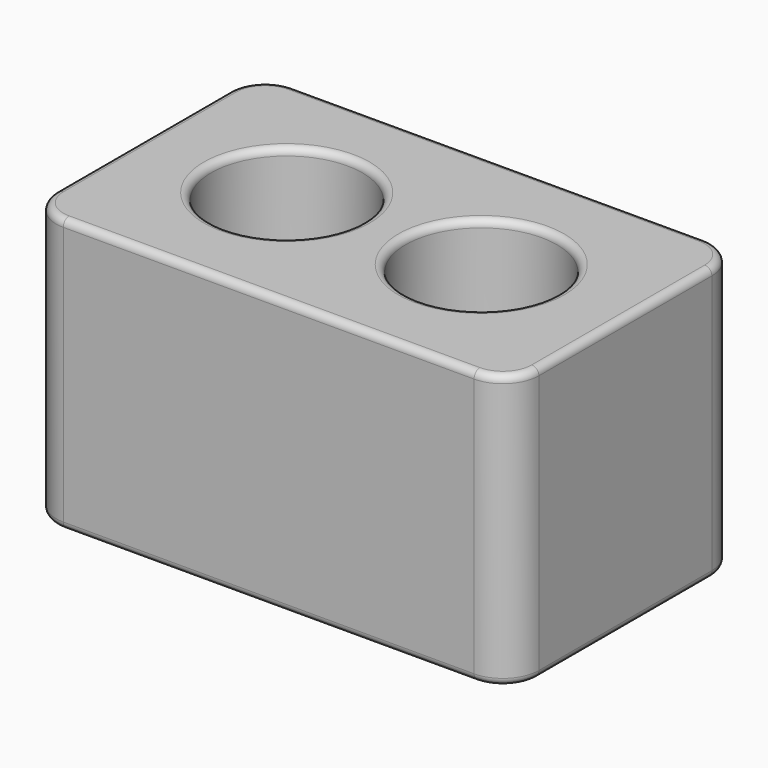
from build123d import *

# Parameters (mm, degrees)
F0_W         = 67
F0_H         = 40
F0_R         = 10.5
F1_DEPTH     = 36
F2_W         = 67
F2_H         = 40
F3_DEPTH     = 2
F4_R         = 1
F5_T1_DEPTH  = 38
F5_T4_ANGLE  = 90
F5_T6_ANGLE  = 90
F5_T8_ANGLE  = 90
F5_T10_ANGLE = 90
F5_T12_ANGLE = 90
F5_T14_ANGLE = 90
F5_T16_ANGLE = 90
F5_T18_ANGLE = 90


# Not quite as in the source:
# - a fillet or chamfer that OpenCascade refuses, or shapes differently, is made with other operations: its cross-section is extruded or revolved along the edge and cut away or added


with BuildPart() as f1:
    # F0 (on Top) → F1 (new body)
    with BuildSketch(Plane.XY):
        Rectangle(F0_W, F0_H)
        with Locations((-13.5, 0)):
            Circle(F0_R, mode=Mode.SUBTRACT)
        with Locations((13.5, 0)):
            Circle(F0_R, mode=Mode.SUBTRACT)
    extrude(amount=F1_DEPTH)

    # F2 (on face) → F3 (join)
    with BuildSketch(Plane(origin=(0, 0, 0), x_dir=(1, 0, 0), z_dir=(0, 0, -1))):
        Rectangle(F2_W, F2_H)
    extrude(amount=F3_DEPTH)

    # F4
    f4_edges = [f1.edges().sort_by_distance(p)[0] for p in [
        (0, 20, 36),
        (-33.5, 0, 36),
        (0, -20, 36),
        (33.5, 0, 36),
        (-24, 0, 36),
        (3, 0, 36),
        (0, 20, -2),
        (33.5, 0, -2),
        (0, -20, -2),
        (-33.5, 0, -2),
    ]]
    fillet(f4_edges, radius=F4_R)

    # F5: fillet of radius 5 on 4 edges, made by hand

    # F5_s2 → F5_t1 (cut)
    with BuildSketch(Plane.XY.offset(-2)):
        with BuildLine():
            ThreePointArc((28.5, 20), (32.0355339059, 18.5355339059), (33.5, 15))
            Line((33.5, 15), (33.5, 20))
            Line((33.5, 20), (28.5, 20))
        make_face()
        with BuildLine():
            ThreePointArc((33.5, -15), (32.0355339059, -18.5355339059), (28.5, -20))
            Line((28.5, -20), (33.5, -20))
            Line((33.5, -20), (33.5, -15))
        make_face()
        with BuildLine():
            ThreePointArc((-33.5, -15), (-32.0355339059, -18.5355339059), (-28.5, -20))
            Line((-28.5, -20), (-33.5, -20))
            Line((-33.5, -20), (-33.5, -15))
        make_face()
        with BuildLine():
            ThreePointArc((-28.5, 20), (-32.0355339059, 18.5355339059), (-33.5, 15))
            Line((-33.5, 15), (-33.5, 20))
            Line((-33.5, 20), (-28.5, 20))
        make_face()
    extrude(amount=F5_T1_DEPTH, mode=Mode.SUBTRACT)

    # F5_s3 → F5_t4 (revolve, cut)
    with BuildSketch(Plane.XZ.offset(-15)):
        with BuildLine():
            ThreePointArc((-32.5, -2), (-33.2071067812, -1.7071067812), (-33.5, -1))
            Line((-33.5, -1), (-33.5, -2))
            Line((-33.5, -2), (-32.5, -2))
        make_face()
    revolve(axis=Axis((-28.5, 15, -2), (0, 0, -1)), revolution_arc=F5_T4_ANGLE, mode=Mode.SUBTRACT)

    # F5_s5 → F5_t6 (revolve, cut)
    with BuildSketch(Plane.YZ.offset(-28.5)):
        with BuildLine():
            ThreePointArc((19, 36), (19.7071067812, 35.7071067812), (20, 35))
            Line((20, 35), (20, 36))
            Line((20, 36), (19, 36))
        make_face()
    revolve(axis=Axis((-28.5, 15, 36), (0, 0, 1)), revolution_arc=F5_T6_ANGLE, mode=Mode.SUBTRACT)

    # F5_s7 → F5_t8 (revolve, cut)
    with BuildSketch(Plane.YZ.offset(-28.5)):
        with BuildLine():
            ThreePointArc((-19, -2), (-19.7071067812, -1.7071067812), (-20, -1))
            Line((-20, -1), (-20, -2))
            Line((-20, -2), (-19, -2))
        make_face()
    revolve(axis=Axis((-28.5, -15, -2), (0, 0, -1)), revolution_arc=F5_T8_ANGLE, mode=Mode.SUBTRACT)

    # F5_s9 → F5_t10 (revolve, cut)
    with BuildSketch(Plane.XZ.offset(15)):
        with BuildLine():
            ThreePointArc((-32.5, 36), (-33.2071067812, 35.7071067812), (-33.5, 35))
            Line((-33.5, 35), (-33.5, 36))
            Line((-33.5, 36), (-32.5, 36))
        make_face()
    revolve(axis=Axis((-28.5, -15, 36), (0, 0, 1)), revolution_arc=F5_T10_ANGLE, mode=Mode.SUBTRACT)

    # F5_s11 → F5_t12 (revolve, cut)
    with BuildSketch(Plane.YZ.offset(28.5)):
        with BuildLine():
            ThreePointArc((-19, 36), (-19.7071067812, 35.7071067812), (-20, 35))
            Line((-20, 35), (-20, 36))
            Line((-20, 36), (-19, 36))
        make_face()
    revolve(axis=Axis((28.5, -15, 36), (0, 0, 1)), revolution_arc=F5_T12_ANGLE, mode=Mode.SUBTRACT)

    # F5_s13 → F5_t14 (revolve, cut)
    with BuildSketch(Plane.XZ.offset(15)):
        with BuildLine():
            ThreePointArc((32.5, -2), (33.2071067812, -1.7071067812), (33.5, -1))
            Line((33.5, -1), (33.5, -2))
            Line((33.5, -2), (32.5, -2))
        make_face()
    revolve(axis=Axis((28.5, -15, -2), (0, 0, -1)), revolution_arc=F5_T14_ANGLE, mode=Mode.SUBTRACT)

    # F5_s15 → F5_t16 (revolve, cut)
    with BuildSketch(Plane.XZ.offset(-15)):
        with BuildLine():
            ThreePointArc((32.5, 36), (33.2071067812, 35.7071067812), (33.5, 35))
            Line((33.5, 35), (33.5, 36))
            Line((33.5, 36), (32.5, 36))
        make_face()
    revolve(axis=Axis((28.5, 15, 36), (0, 0, 1)), revolution_arc=F5_T16_ANGLE, mode=Mode.SUBTRACT)

    # F5_s17 → F5_t18 (revolve, cut)
    with BuildSketch(Plane.YZ.offset(28.5)):
        with BuildLine():
            ThreePointArc((19, -2), (19.7071067812, -1.7071067812), (20, -1))
            Line((20, -1), (20, -2))
            Line((20, -2), (19, -2))
        make_face()
    revolve(axis=Axis((28.5, 15, -2), (0, 0, -1)), revolution_arc=F5_T18_ANGLE, mode=Mode.SUBTRACT)


solid = f1.part
